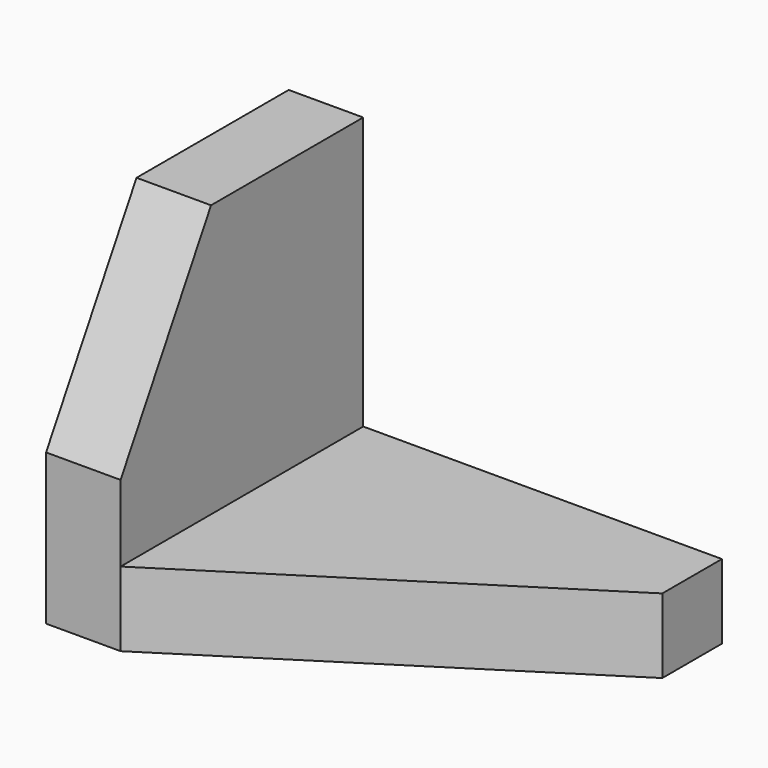
from build123d import *

# Parameters (mm, degrees)
F1_DEPTH = 10.922
F3_DEPTH = 33.528
F5_DEPTH = 25.4
F7_DEPTH = 25.4


# Not quite as in the source:
# - a feature names something its author has since deleted; it is built from what else it names


with BuildPart() as f1:
    # F0 (on Front) → F1 (new body)
    with BuildSketch(Plane.XZ):
        Polygon((0, 50.8), (0, 0), (63.5, 0), (63.5, 10.922), (10.922, 10.922), (10.922, 50.8), align=None)
    extrude(amount=F1_DEPTH)

    # F2 (on face) → F3 (join)
    with BuildSketch(Plane.XZ.offset(10.922)):
        Polygon((0, 10.922), (0, 0), (10.922, 0), (63.5, 0), (63.5, 10.922), (10.922, 10.922), (10.922, 50.8), (0, 50.8), align=None)
    extrude(amount=F3_DEPTH)

    # F4 (on face) → F5 (cut)
    with BuildSketch(Plane.XY.offset(10.922)):
        Polygon((63.5, -10.922), (10.922, -44.45), (63.5, -44.45), align=None)
    extrude(amount=-F5_DEPTH, mode=Mode.SUBTRACT)

    # F6 (on face) → F7 (cut)
    with BuildSketch(Plane(origin=(0, 0, 0), x_dir=(0, -1, 0), z_dir=(-1, 0, 0))):
        Polygon((27.8788925737, 50.8), (44.45, 22.098), (44.45, 50.8), align=None)
    extrude(amount=-F7_DEPTH, mode=Mode.SUBTRACT)


solid = f1.part
